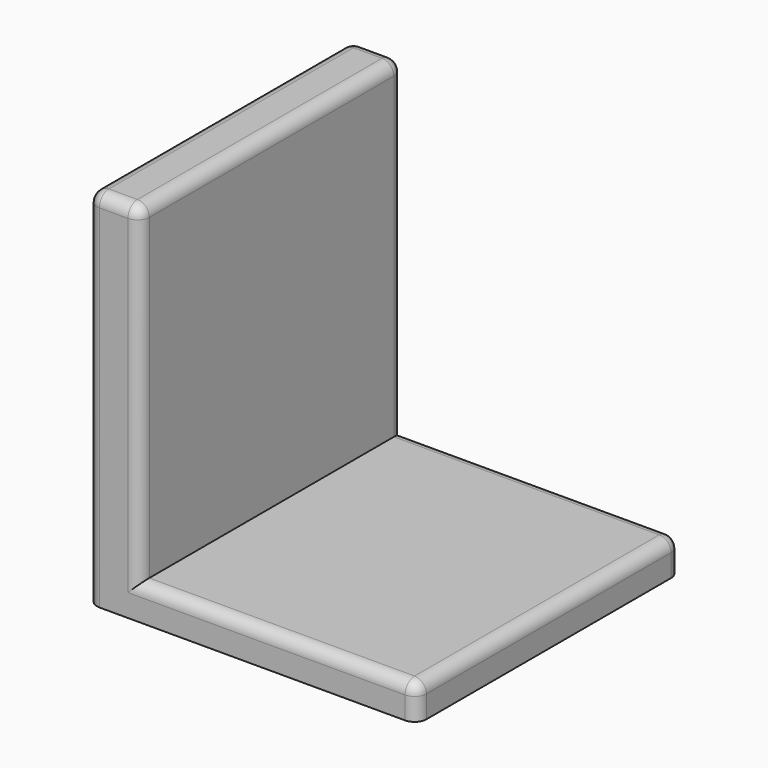
from build123d import *

# Parameters (mm, degrees)
F0_W         = 503.2831068337
F0_H         = 635
F0_W_2       = 131.7168931663
F1_DEPTH     = 66.04
F2_W         = 100.6971086562
F2_H         = 635
F3_DEPTH     = 635
F4_R         = 22.86
F5_R         = 22.86
F6_R         = 22.86
F7_T1_DEPTH  = 100.33
F7_S5_W      = 22.86
F7_S5_H      = 22.86
F7_T6_DEPTH  = 22.86
F7_S11_W     = 22.86
F7_S11_H     = 22.86
F7_T12_DEPTH = 22.86


# Not quite as in the source:
# - a fillet or chamfer that OpenCascade refuses, or shapes differently, is made with other operations: its cross-section is extruded or revolved along the edge and cut away or added


with BuildPart() as f1:
    # F0 (on Top) → F1 (new body)
    with BuildSketch(Plane.XY):
        with Locations((-52.821796909, 15.8370759291)):
            Rectangle(F0_W, F0_H)
        with Locations((264.678203091, 15.8370759291)):
            Rectangle(F0_W_2, F0_H)
    extrude(amount=F1_DEPTH)

    # F2 (on face) → F3 (join)
    with BuildSketch(Plane.XY.offset(66.04)):
        with Locations((-254.1147959977, 15.8370759291)):
            Rectangle(F2_W, F2_H)
    extrude(amount=F3_DEPTH)

    # F4
    f4_edges = [f1.edges().sort_by_distance(p)[0] for p in [
        (-203.766242, 15.837076, 701.04),
        (-304.46335, 15.837076, 701.04),
    ]]
    fillet(f4_edges, radius=F4_R)

    # F5
    f5_edges = [f1.edges().sort_by_distance(p)[0] for p in [
        (-203.766242, -301.662924, 372.11),
        (63.385204, -301.662924, 66.04),
        (330.53665, 15.837076, 66.04),
        (63.385204, 333.337076, 66.04),
    ]]
    fillet(f5_edges, radius=F5_R)

    # F6
    f6_edges = [f1.edges().sort_by_distance(p)[0] for p in [
        (-203.766242, 333.337076, 372.11),
        (-304.46335, 333.337076, 339.09),
    ]]
    fillet(f6_edges, radius=F6_R)

    # F7: fillet of radius 22.86 on 2 edges, made by hand

    # F7_s2 → F7_t1 (cut)
    with BuildSketch(Plane.XY.offset(-57.15)):
        with BuildLine():
            ThreePointArc((307.6766496742, 333.3370759291), (323.8411106921, 326.641536947), (330.5366496742, 310.4770759291))
            Line((330.5366496742, 310.4770759291), (330.5366496742, 333.3370759291))
            Line((330.5366496742, 333.3370759291), (307.6766496742, 333.3370759291))
        make_face()
        with BuildLine():
            ThreePointArc((307.6766496742, -301.6629240709), (323.8411106921, -294.9673850888), (330.5366496742, -278.8029240709))
            Line((330.5366496742, -278.8029240709), (330.5366496742, -301.6629240709))
            Line((330.5366496742, -301.6629240709), (307.6766496742, -301.6629240709))
        make_face()
    extrude(amount=F7_T1_DEPTH, mode=Mode.SUBTRACT)


with BuildPart() as f7_tool4:
    # F7_s5 → F7_t6 (new body)
    with BuildSketch(Plane.XZ.offset(278.8029240709)):
        with Locations((319.1066496742, 54.61)):
            Rectangle(F7_S5_W, F7_S5_H)
    extrude(amount=F7_T6_DEPTH)

    # F7_s7 → F7_t8 (revolve, cut)
    with BuildSketch(Plane(origin=(307.6766496742, -278.8029240709, 43.18), x_dir=(-0.7071067812, 0, -0.7071067812), z_dir=(-0.7071067812, 0, 0.7071067812))):
        with BuildLine():
            ThreePointArc((0, -22.86), (22.86, 0), (0, 22.86))
            Line((0, 22.86), (0, -22.86))
        make_face()
    revolve(axis=Axis((307.6766496742, -278.8029240709, 43.18), (0, -1, 0)), mode=Mode.SUBTRACT)


with BuildPart() as f1_1:
    add(f1.part)

    # F7_t3: cut F7_tool4
    add(f7_tool4.part, mode=Mode.SUBTRACT)


with BuildPart() as f7_tool10:
    # F7_s11 → F7_t12 (new body)
    with BuildSketch(Plane.XZ.offset(-310.4770759291)):
        with Locations((319.1066496742, 54.61)):
            Rectangle(F7_S11_W, F7_S11_H)
    extrude(amount=-F7_T12_DEPTH)

    # F7_s13 → F7_t14 (revolve, cut)
    with BuildSketch(Plane(origin=(307.6766496742, 310.4770759291, 43.18), x_dir=(-0.7071067812, 0, -0.7071067812), z_dir=(0.7071067812, 0, -0.7071067812))):
        with BuildLine():
            ThreePointArc((0, -22.86), (22.86, 0), (0, 22.86))
            Line((0, 22.86), (0, -22.86))
        make_face()
    revolve(axis=Axis((307.6766496742, 310.4770759291, 43.18), (0, 1, 0)), mode=Mode.SUBTRACT)


with BuildPart() as f1_2:
    add(f1_1.part)

    # F7_t9: cut F7_tool10
    add(f7_tool10.part, mode=Mode.SUBTRACT)


solid = f1_2.part
